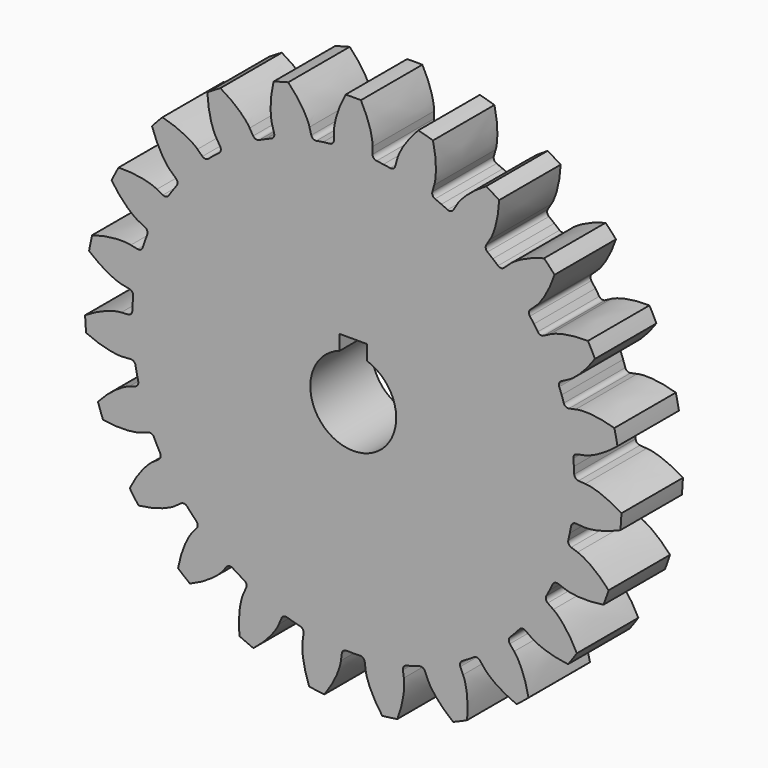
from build123d import *

# Parameters (mm, degrees)
F0_R     = 762
F1_DEPTH = 431.8


# Not quite as in the source:
# - ends of sketch curves that miss each other by under 0.0002 mm in the source are joined
# - the dataset's text gives a spline's control points without its knots; the knots are read off the source's solid


with BuildPart() as f1:
    # F0 (on Front) → F1 (new body)
    with BuildSketch(Plane.XZ):
        with BuildLine():
            ThreePointArc((207.1917137632, 1220.8943197928), (188.2251520352, 1223.9508569959), (169.2136060356, 1226.7138268041))
            ThreePointArc((169.2136060356, 1226.7138268041), (150.1616235918, 1229.1825683762), (131.0737537642, 1231.3564923478))
            ThreePointArc((131.0737537642, 1231.3564923478), (114.8688538687, 1239.6278770922), (108.3528186, 1256.6148096))
            Line((108.3528186, 1256.6148096), (108.3528186, 1294.8832116))
            add(Edge.make_bspline(
                [(42.8680118, 1503.1089826), (49.4976658, 1490.9197258), (64.0712968, 1462.3371058), (82.4042802, 1419.0365828), (96.2182734, 1376.5073308), (104.123363, 1342.6242388), (107.5962542, 1318.038004), (108.630847, 1303.1525118), (108.4084446, 1296.537158), (108.3528186, 1294.8832116)],
                knots=[7.154307, 7.154307, 7.154307, 7.154307, 8.792592, 10.941893, 12.700413, 14.068152, 15.04511, 15.631289, 15.826701, 15.826701, 15.826701, 15.826701], degree=3))
            ThreePointArc((42.8680118, 1503.1089826), (0, 1503.718354), (-42.8680115994, 1503.1089755464))
            add(Edge.make_bspline(
                [(-42.8680115994, 1503.1089755464), (-49.4976658, 1490.9197258), (-64.0712968, 1462.3371058), (-82.4042802, 1419.0365828), (-96.2182734, 1376.5073308), (-104.123363, 1342.6242388), (-107.5962542, 1318.038004), (-108.630847, 1303.1525118), (-108.4084446, 1296.537158), (-108.3528186, 1294.8832116)],
                knots=[7.154307, 7.154307, 7.154307, 7.154307, 8.792592, 10.941893, 12.700413, 14.068152, 15.04511, 15.631289, 15.826701, 15.826701, 15.826701, 15.826701], degree=3))
            Line((-108.3528186, 1294.8832116), (-108.3528186, 1256.6148096))
            ThreePointArc((-108.3528186, 1256.6148096), (-114.8688538687, 1239.6278770922), (-131.0737537202, 1231.3564919329))
            ThreePointArc((-131.0737537202, 1231.3564919329), (-150.1616235918, 1229.1825683762), (-169.2136060356, 1226.7138268041))
            ThreePointArc((-169.2136060356, 1226.7138268041), (-188.2251520352, 1223.9508569959), (-207.1917137632, 1220.8943197928))
            ThreePointArc((-207.1917137632, 1220.8943197928), (-225.0272880967, 1224.4869450629), (-235.884706456, 1239.0859614781))
            Line((-235.884706456, 1239.0859614781), (-246.2093882, 1275.9352688))
            add(Edge.make_bspline(
                [(-365.4445066, 1458.7718602), (-355.7720596, 1448.8232898), (-334.0273482, 1425.2325064), (-304.6918976, 1388.4838626), (-279.9158994, 1351.258664), (-263.1623896, 1320.764821), (-253.1850156, 1298.0272998), (-248.1727066, 1283.972921), (-246.6020722, 1277.5428856), (-246.2093882, 1275.9352688)],
                knots=[7.154307, 7.154307, 7.154307, 7.154307, 8.792592, 10.941893, 12.700413, 14.068152, 15.04511, 15.631289, 15.826701, 15.826701, 15.826701, 15.826701], degree=3))
            ThreePointArc((-365.4445066, 1458.7718602), (-406.8872538926, 1447.7929884321), (-448.001185685, 1435.6405592158))
            add(Edge.make_bspline(
                [(-448.001185685, 1435.6405592158), (-451.0964054, 1422.1146564), (-457.4181098, 1390.660033), (-463.3888878, 1344.019029), (-465.216367, 1299.339921), (-463.686779, 1264.580529), (-460.3975806, 1239.969072), (-457.3777746, 1225.3564266), (-455.3787946, 1219.0463808), (-454.8790242, 1217.4687614)],
                knots=[7.154307, 7.154307, 7.154307, 7.154307, 8.792592, 10.941893, 12.700413, 14.068152, 15.04511, 15.631289, 15.826701, 15.826701, 15.826701, 15.826701], degree=3))
            Line((-454.8790242, 1217.4687614), (-444.5543306, 1180.6194574))
            ThreePointArc((-444.5543306, 1180.6194574), (-446.2457074648, 1162.5044593237), (-459.6180792046, 1150.1677764018))
            ThreePointArc((-459.6180792046, 1150.1677764018), (-477.4116048133, 1142.924615064), (-495.0910348076, 1135.4072555989))
            ThreePointArc((-495.0910348076, 1135.4072555989), (-512.6521460867, 1127.6174880792), (-530.0907376222, 1119.5571758876))
            ThreePointArc((-530.0907376222, 1119.5571758876), (-548.2341895487, 1118.2046140224), (-562.6277429952, 1129.332952857))
            Line((-562.6277429952, 1129.332952857), (-582.5113826, 1162.0302134))
            add(Edge.make_bspline(
                [(-746.6536756, 1305.9174796), (-734.6558078, 1298.9474148), (-707.3527382, 1282.0980962), (-669.190432, 1254.6268024), (-635.2899918, 1225.4665102), (-610.9306044, 1200.6235068), (-595.1887004, 1181.4210306), (-586.570455, 1169.2401304), (-583.3232428, 1163.472273), (-582.5113826, 1162.0302134)],
                knots=[7.154307, 7.154307, 7.154307, 7.154307, 8.792592, 10.941893, 12.700413, 14.068152, 15.04511, 15.631289, 15.826701, 15.826701, 15.826701, 15.826701], degree=3))
            ThreePointArc((-746.6536756, 1305.9174796), (-783.5975441911, 1284.1646187591), (-819.9081683383, 1261.3704319712))
            add(Edge.make_bspline(
                [(-819.9081683383, 1261.3704319712), (-819.2393572, 1247.5110178), (-816.8402764, 1215.517254), (-810.0060762, 1168.9949442), (-799.7114816, 1125.479588), (-788.8606524, 1092.4218436), (-779.0533314, 1069.6104592), (-772.203053, 1056.3544278), (-768.575806, 1050.8177104), (-767.6689244, 1049.4334358)],
                knots=[7.154307, 7.154307, 7.154307, 7.154307, 8.792592, 10.941893, 12.700413, 14.068152, 15.04511, 15.631289, 15.826701, 15.826701, 15.826701, 15.826701], degree=3))
            Line((-767.6689244, 1049.4334358), (-747.785271, 1016.7361682))
            ThreePointArc((-747.785271, 1016.7361682), (-744.5265483812, 998.8365845229), (-754.0746415401, 983.3495450455))
            ThreePointArc((-754.0746415401, 983.3495450455), (-769.2541625123, 971.5743458654), (-784.2498366521, 959.5658934098))
            ThreePointArc((-784.2498366521, 959.5658934098), (-799.0580687681, 947.3270697848), (-813.6753327189, 934.8607897976))
            ThreePointArc((-813.6753327189, 934.8607897976), (-830.7810656895, 928.6633348644), (-847.6432640421, 935.49566387))
            Line((-847.6432640421, 935.49566387), (-875.6111774, 961.6158822))
            add(Edge.make_bspline(
                [(-1072.486933, 1055.8823688), (-1059.053508, 1052.4077504), (-1028.217019, 1043.5495258), (-984.0582046, 1027.3930176), (-943.547516, 1008.4602894), (-913.3888768, 991.1106162), (-893.0499538, 976.8673122), (-881.4649376, 967.4632924), (-876.7820158, 962.7854252), (-875.6111774, 961.6158822)],
                knots=[7.154307, 7.154307, 7.154307, 7.154307, 8.792592, 10.941893, 12.700413, 14.068152, 15.04511, 15.631289, 15.826701, 15.826701, 15.826701, 15.826701], degree=3))
            ThreePointArc((-1072.486933, 1055.8823688), (-1102.1919871804, 1024.9688146655), (-1131.0063300048, 993.2233942023))
            add(Edge.make_bspline(
                [(-1131.0063300048, 993.2233942023), (-1126.623096, 980.0583904), (-1115.681157, 949.8983034), (-1096.5488102, 906.9449984), (-1074.8956658, 867.8207688), (-1055.5283436, 838.916407), (-1039.9302798, 819.596913), (-1029.7575798, 808.680628), (-1024.7710518, 804.3278554), (-1023.5243182, 803.2395924)],
                knots=[7.154307, 7.154307, 7.154307, 7.154307, 8.792592, 10.941893, 12.700413, 14.068152, 15.04511, 15.631289, 15.826701, 15.826701, 15.826701, 15.826701], degree=3))
            Line((-1023.5243182, 803.2395924), (-995.5564036, 777.1193754))
            ThreePointArc((-995.5564036, 777.1193754), (-987.5892794345, 760.7627410412), (-992.6049562675, 743.2739570743))
            ThreePointArc((-992.6049562675, 743.2739570743), (-1004.0446531194, 727.8400320856), (-1015.244398185, 712.2311111541))
            ThreePointArc((-1015.244398185, 712.2311111541), (-1026.2015132755, 696.4509124069), (-1036.9133744925, 680.5032143638))
            ThreePointArc((-1036.9133744925, 680.5032143638), (-1051.7127205279, 669.9205067122), (-1069.7929606689, 671.9501118353))
            Line((-1069.7929606689, 671.9501118353), (-1103.7709192, 689.5560758))
            add(Edge.make_bspline(
                [(-1318.7787696, 727.2104582), (-1304.9060262, 727.4889946), (-1272.8231338, 727.278835), (-1225.9428872, 723.6353574), (-1181.82644, 716.334356), (-1148.1052984, 707.764777), (-1124.6777862, 699.5370312), (-1110.985205, 693.6073504), (-1105.2138424, 690.3663612), (-1103.7709192, 689.5560758)],
                knots=[7.154307, 7.154307, 7.154307, 7.154307, 8.792592, 10.941893, 12.700413, 14.068152, 15.04511, 15.631289, 15.826701, 15.826701, 15.826701, 15.826701], degree=3))
            ThreePointArc((-1318.7787696, 727.2104582), (-1339.0418965789, 689.4289359871), (-1358.2229115881, 651.0867087047))
            add(Edge.make_bspline(
                [(-1358.2229115881, 651.0867087047), (-1350.4503344, 639.5924724), (-1331.7770672, 613.5029132), (-1301.7655194, 577.304281), (-1270.3597656, 545.4728232), (-1243.9123204, 522.8655786), (-1223.6803314, 508.470789), (-1210.9397168, 500.7038754), (-1204.9637064, 497.8578562), (-1203.4696022, 497.146326)],
                knots=[7.154307, 7.154307, 7.154307, 7.154307, 8.792592, 10.941893, 12.700413, 14.068152, 15.04511, 15.631289, 15.826701, 15.826701, 15.826701, 15.826701], degree=3))
            Line((-1203.4696022, 497.146326), (-1169.4916666, 479.5403668))
            ThreePointArc((-1169.4916666, 479.5403668), (-1157.4070195713, 465.9397877294), (-1157.5182855896, 447.7463236647))
            ThreePointArc((-1157.5182855896, 447.7463236647), (-1164.3697442422, 429.7983306164), (-1170.9429379142, 411.7465699841))
            ThreePointArc((-1170.9429379142, 411.7465699841), (-1177.2362828369, 393.5953607754), (-1183.248278145, 375.3490324195))
            ThreePointArc((-1183.248278145, 375.3490324195), (-1194.6436427881, 361.1659361482), (-1212.6010042574, 358.242283599))
            Line((-1212.6010042574, 358.242283599), (-1250.0689756, 366.028224))
            add(Edge.make_bspline(
                [(-1467.2628008, 344.2778484), (-1453.9796676, 348.2888894), (-1423.0297676, 356.7423904), (-1376.9049678, 365.8821486), (-1332.4547138, 370.7543766), (-1297.6719792, 371.6004252), (-1272.8934156, 369.9984472), (-1258.1087614, 367.9828556), (-1251.6770242, 366.4191808), (-1250.0689756, 366.028224)],
                knots=[7.154307, 7.154307, 7.154307, 7.154307, 8.792592, 10.941893, 12.700413, 14.068152, 15.04511, 15.631289, 15.826701, 15.826701, 15.826701, 15.826701], degree=3))
            ThreePointArc((-1467.2628008, 344.2778484), (-1476.5811900429, 302.4304522076), (-1484.7063103238, 260.3350917556))
            add(Edge.make_bspline(
                [(-1484.7063103238, 260.3350917556), (-1474.1208516, 251.364115), (-1449.1011658, 231.2800048), (-1410.4362698, 204.5207238), (-1371.6070866, 182.3428408), (-1340.0410334, 167.709342), (-1316.6756242, 159.306895), (-1302.311975, 155.2653994), (-1295.7897376, 154.1372076), (-1294.1590576, 153.855166)],
                knots=[7.154307, 7.154307, 7.154307, 7.154307, 8.792592, 10.941893, 12.700413, 14.068152, 15.04511, 15.631289, 15.826701, 15.826701, 15.826701, 15.826701], degree=3))
            Line((-1294.1590576, 153.855166), (-1256.6910858, 146.0692278))
            ThreePointArc((-1256.6910858, 146.0692278), (-1241.385179011, 136.233393155), (-1236.5837786479, 118.6845752562))
            ThreePointArc((-1236.5837786479, 118.6845752562), (-1238.3388559954, 99.5536385174), (-1239.7979913123, 80.3978572005))
            ThreePointArc((-1239.7979913123, 80.3978572005), (-1240.9608244985, 61.221816461), (-1241.8270783309, 42.0300910628))
            ThreePointArc((-1241.8270783309, 42.0300910628), (-1248.9733177093, 25.298515831), (-1265.4759809502, 17.6384509204))
            Line((-1265.4759809502, 17.6384509204), (-1303.6551778, 15.0269194))
            add(Edge.make_bspline(
                [(-1506.9266788, -64.5150856), (-1495.2182694, -57.0690502), (-1467.6968106, -40.5788368), (-1425.7483296, -19.3336672), (-1384.2609094, -2.649601), (-1350.996282, 7.5493626), (-1326.704357, 12.6919482), (-1311.9241732, 14.7399756), (-1305.3090734, 14.9695154), (-1303.6551778, 15.0269194)],
                knots=[7.154307, 7.154307, 7.154307, 7.154307, 8.792592, 10.941893, 12.700413, 14.068152, 15.04511, 15.631289, 15.826701, 15.826701, 15.826701, 15.826701], degree=3))
            ThreePointArc((-1506.9266788, -64.5150856), (-1504.6092126713, -107.3247336701), (-1501.0758396072, -150.0512112007))
            add(Edge.make_bspline(
                [(-1501.0758396072, -150.0512112007), (-1488.4625806, -155.8336228), (-1458.9520478, -168.4227264), (-1414.5013874, -183.7580272), (-1371.128576, -194.6375076), (-1336.7850074, -200.2119186), (-1312.0191184, -201.9988848), (-1297.0977106, -202.0152424), (-1290.5129638, -201.3419138), (-1288.8666628, -201.1735626)],
                knots=[7.154307, 7.154307, 7.154307, 7.154307, 8.792592, 10.941893, 12.700413, 14.068152, 15.04511, 15.631289, 15.826701, 15.826701, 15.826701, 15.826701], degree=3))
            Line((-1288.8666628, -201.1735626), (-1250.6874656, -198.5620362))
            ThreePointArc((-1250.6874656, -198.5620362), (-1233.2954715893, -203.903634229), (-1223.9375104416, -219.5062927103))
            ThreePointArc((-1223.9375104416, -219.5062927103), (-1220.4660423092, -238.4013096037), (-1216.7029025722, -257.2404054098))
            ThreePointArc((-1216.7029025722, -257.2404054098), (-1212.6489780375, -276.0190888106), (-1208.3052400256, -294.7328589942))
            ThreePointArc((-1208.3052400256, -294.7328589942), (-1210.6723585001, -312.7720099861), (-1224.4963843289, -324.6003873353))
            Line((-1224.4963843289, -324.6003873353), (-1260.5552132, -337.4156828))
            add(Edge.make_bspline(
                [(-1434.8286772, -468.8500402), (-1425.5633668, -458.5212318), (-1403.5114932, -435.2173414), (-1368.85045, -403.442424), (-1333.4028196, -376.1838806), (-1304.1233506, -357.3884394), (-1282.1197116, -345.8826712), (-1268.4401606, -339.9229422), (-1262.1322992, -337.9171804), (-1260.5552132, -337.4156828)],
                knots=[7.154307, 7.154307, 7.154307, 7.154307, 8.792592, 10.941893, 12.700413, 14.068152, 15.04511, 15.631289, 15.826701, 15.826701, 15.826701, 15.826701], degree=3))
            ThreePointArc((-1434.8286772, -468.8500402), (-1421.0472548272, -509.4469564436), (-1406.1174406458, -549.6357343076))
            add(Edge.make_bspline(
                [(-1406.1174406458, -549.6357343076), (-1392.4118456, -551.8006744), (-1360.5991584, -555.9611182), (-1313.659425, -558.735103), (-1268.959743, -557.509299), (-1234.385771, -553.6112118), (-1210.056127, -548.6501346), (-1195.6836386, -544.6401604), (-1189.5247482, -542.2152478), (-1187.9848986, -541.6089752)],
                knots=[7.154307, 7.154307, 7.154307, 7.154307, 8.792592, 10.941893, 12.700413, 14.068152, 15.04511, 15.631289, 15.826701, 15.826701, 15.826701, 15.826701], degree=3))
            Line((-1187.9848986, -541.6089752), (-1151.9260934, -528.7936592))
            ThreePointArc((-1151.9260934, -528.7936592), (-1133.7378843182, -529.2448847468), (-1120.5173863074, -541.7442014947))
            ThreePointArc((-1120.5173863074, -541.7442014947), (-1112.0768418425, -559.0019586944), (-1103.3705195132, -576.127171864))
            ThreePointArc((-1103.3705195132, -576.127171864), (-1094.4005004888, -593.1157486601), (-1085.1689286269, -609.9636287587))
            ThreePointArc((-1085.1689286269, -609.9636287587), (-1082.5813731463, -627.9724758858), (-1092.7015046064, -643.0918966742))
            Line((-1092.7015046064, -643.0918966742), (-1123.9656464, -665.1605442))
            add(Edge.make_bspline(
                [(-1256.316004, -838.739369), (-1250.1809642, -826.2938262), (-1235.2341564, -797.9045764), (-1210.4311834, -757.9565232), (-1183.652319, -722.1451394), (-1160.5295814, -696.147198), (-1142.4461022, -679.1315602), (-1130.8817362, -669.7021404), (-1125.3489304, -666.068899), (-1123.9656464, -665.1605442)],
                knots=[7.154307, 7.154307, 7.154307, 7.154307, 8.792592, 10.941893, 12.700413, 14.068152, 15.04511, 15.631289, 15.826701, 15.826701, 15.826701, 15.826701], degree=3))
            ThreePointArc((-1256.316004, -838.739369), (-1232.0927158282, -874.1126625528), (-1206.8737342356, -908.7831191776))
            add(Edge.make_bspline(
                [(-1206.8737342356, -908.7831191776), (-1193.0922798, -907.1700424), (-1161.3368188, -902.5932418), (-1115.3893364, -892.6001706), (-1072.6779664, -879.3599888), (-1040.4377718, -866.2785062), (-1018.3488396, -854.9373554), (-1005.5911816, -847.1984326), (-1000.3149158, -843.201768), (-998.9957414, -842.202532)],
                knots=[7.154307, 7.154307, 7.154307, 7.154307, 8.792592, 10.941893, 12.700413, 14.068152, 15.04511, 15.631289, 15.826701, 15.826701, 15.826701, 15.826701], degree=3))
            Line((-998.9957414, -842.202532), (-967.731618, -820.1338944))
            ThreePointArc((-967.731618, -820.1338944), (-950.0961395823, -815.6612726178), (-933.9936239178, -824.1302434205))
            ThreePointArc((-933.9936239178, -824.1302434205), (-921.2099913722, -838.4708010991), (-908.2061979962, -852.6120249892))
            ThreePointArc((-908.2061979962, -852.6120249892), (-894.9853513159, -866.5505341967), (-881.5506104913, -880.2829980997))
            ThreePointArc((-881.5506104913, -880.2829980997), (-874.2002628674, -896.9259218018), (-879.8659530492, -914.2150656515))
            Line((-879.8659530492, -914.2150656515), (-904.0166832, -943.9002966))
            add(Edge.make_bspline(
                [(-984.6281298, -1146.750056), (-982.0783508, -1133.1108148), (-975.345141, -1101.7417132), (-962.2397824, -1056.5832818), (-946.1157608, -1014.875034), (-930.8646356, -983.6027064), (-918.0425124, -962.339198), (-909.4510132, -950.1394256), (-905.1036, -945.1481986), (-904.0166832, -943.9002966)],
                knots=[7.154307, 7.154307, 7.154307, 7.154307, 8.792592, 10.941893, 12.700413, 14.068152, 15.04511, 15.631289, 15.826701, 15.826701, 15.826701, 15.826701], degree=3))
            ThreePointArc((-984.6281298, -1146.750056), (-951.7595055841, -1174.2762366618), (-918.121739889, -1200.8570153711))
            add(Edge.make_bspline(
                [(-918.121739889, -1200.8570153711), (-905.2865308, -1195.5855692), (-875.9434602, -1182.6109698), (-834.3959436, -1160.5919892), (-796.8405704, -1136.3193936), (-769.3252838, -1115.0247194), (-751.1152618, -1098.1445906), (-740.918635, -1087.250683), (-736.9163062, -1081.9787098), (-735.9156478, -1080.6606276)],
                knots=[7.154307, 7.154307, 7.154307, 7.154307, 8.792592, 10.941893, 12.700413, 14.068152, 15.04511, 15.631289, 15.826701, 15.826701, 15.826701, 15.826701], degree=3))
            Line((-735.9156478, -1080.6606276), (-711.7649214, -1050.9753936))
            ThreePointArc((-711.7649214, -1050.9753936), (-695.9901259568, -1041.9106321688), (-678.1998408489, -1045.7211294955))
            ThreePointArc((-678.1998408489, -1045.7211294955), (-662.0212203823, -1056.0809143876), (-645.6843854666, -1066.1893626561))
            ThreePointArc((-645.6843854666, -1066.1893626561), (-629.193233555, -1076.0440557024), (-612.5517095331, -1085.6426360471))
            ThreePointArc((-612.5517095331, -1085.6426360471), (-600.9837283129, -1099.6853020294), (-601.7747607234, -1117.8619025607))
            Line((-601.7747607234, -1117.8619025607), (-617.0209402, -1152.9621086))
            add(Edge.make_bspline(
                [(-639.9148746, -1370.0383572), (-641.1394848, -1356.2169726), (-643.119237, -1324.1945068), (-642.6834746, -1277.1749158), (-638.4101024, -1232.6630922), (-632.1617024, -1198.4357286), (-625.5518858, -1174.5013848), (-620.5704378, -1160.4360332), (-617.7308702, -1154.4569748), (-617.0209402, -1152.9621086)],
                knots=[7.154307, 7.154307, 7.154307, 7.154307, 8.792592, 10.941893, 12.700413, 14.068152, 15.04511, 15.631289, 15.826701, 15.826701, 15.826701, 15.826701], degree=3))
            ThreePointArc((-639.9148746, -1370.0383572), (-600.8386419489, -1387.6759408107), (-561.2768558469, -1404.1956682157))
            add(Edge.make_bspline(
                [(-561.2768558469, -1404.1956682157), (-550.3398188, -1395.6568226), (-525.5853852, -1375.246678), (-491.51921, -1342.8348048), (-461.9051468, -1309.3300204), (-441.1554296, -1281.4014504), (-428.174912, -1260.2343096), (-421.2955506, -1246.9933404), (-418.8639832, -1240.8370408), (-418.2560596, -1239.297877)],
                knots=[7.154307, 7.154307, 7.154307, 7.154307, 8.792592, 10.941893, 12.700413, 14.068152, 15.04511, 15.631289, 15.826701, 15.826701, 15.826701, 15.826701], degree=3))
            Line((-418.2560596, -1239.297877), (-403.0098874, -1204.1976678))
            ThreePointArc((-403.0098874, -1204.1976678), (-390.2656925401, -1191.2130621309), (-372.1070557635, -1190.0824882937))
            ThreePointArc((-372.1070557635, -1190.0824882937), (-353.7333473791, -1195.6931698795), (-335.275099724, -1201.019144067))
            ThreePointArc((-335.275099724, -1201.019144067), (-316.7367201822, -1206.0591386589), (-298.1226431187, -1210.8119479964))
            ThreePointArc((-298.1226431187, -1210.8119479964), (-283.1949670005, -1221.2128578376), (-279.0526829476, -1238.9288400498))
            Line((-279.0526829476, -1238.9288400498), (-284.2635666, -1276.8408042))
            add(Edge.make_bspline(
                [(-247.742075, -1492.0439806), (-252.650244, -1479.0655458), (-263.1961208, -1448.764692), (-275.4622634, -1403.3711328), (-283.3565072, -1359.3569968), (-286.57423, -1324.7130732), (-286.66694, -1299.882973), (-285.6650116, -1284.9952456), (-284.543881, -1278.471789), (-284.2635666, -1276.8408042)],
                knots=[7.154307, 7.154307, 7.154307, 7.154307, 8.792592, 10.941893, 12.700413, 14.068152, 15.04511, 15.631289, 15.826701, 15.826701, 15.826701, 15.826701], degree=3))
            ThreePointArc((-247.742075, -1492.0439806), (-205.3563291936, -1498.4848881564), (-162.8046272215, -1503.7183777557))
            add(Edge.make_bspline(
                [(-162.8046272215, -1503.7183777557), (-154.5769324, -1492.545402), (-136.2470478, -1466.2134506), (-112.1887266, -1425.8125662), (-92.7123622, -1385.5604242), (-80.2671242, -1353.0693284), (-73.478771, -1329.1849972), (-70.4268848, -1314.579032), (-69.7464442, -1307.9949964), (-69.576315, -1306.3488986)],
                knots=[7.154307, 7.154307, 7.154307, 7.154307, 8.792592, 10.941893, 12.700413, 14.068152, 15.04511, 15.631289, 15.826701, 15.826701, 15.826701, 15.826701], degree=3))
            Line((-69.576315, -1306.3488986), (-64.3654288, -1268.4369094))
            ThreePointArc((-64.3654288, -1268.4369094), (-55.5970452045, -1252.4954617702), (-38.4167887865, -1246.5076919647))
            ThreePointArc((-38.4167887865, -1246.5076919647), (-19.2106900217, -1246.9531491193), (0, -1247.101646))
            ThreePointArc((0, -1247.101646), (19.2106900217, -1246.9531491193), (38.4167888485, -1246.5076939665))
            ThreePointArc((38.4167888485, -1246.5076939665), (55.5970452045, -1252.4954617702), (64.3654511814, -1268.4369063237))
            Line((64.3654511814, -1268.4369063237), (69.576315, -1306.3488986))
            add(Edge.make_bspline(
                [(162.8046274, -1503.7183794), (154.5769324, -1492.545402), (136.2470478, -1466.2134506), (112.1887266, -1425.8125662), (92.7123622, -1385.5604242), (80.2671242, -1353.0693284), (73.478771, -1329.1849972), (70.4268848, -1314.579032), (69.7464442, -1307.9949964), (69.576315, -1306.3488986)],
                knots=[7.154307, 7.154307, 7.154307, 7.154307, 8.792592, 10.941893, 12.700413, 14.068152, 15.04511, 15.631289, 15.826701, 15.826701, 15.826701, 15.826701], degree=3))
            ThreePointArc((162.8046274, -1503.7183794), (205.3563291936, -1498.4848881564), (247.7420772114, -1492.0439938788))
            add(Edge.make_bspline(
                [(247.7420772114, -1492.0439938788), (252.650244, -1479.0655458), (263.1961208, -1448.764692), (275.4622634, -1403.3711328), (283.3565072, -1359.3569968), (286.57423, -1324.7130732), (286.66694, -1299.882973), (285.6650116, -1284.9952456), (284.543881, -1278.471789), (284.2635666, -1276.8408042)],
                knots=[7.154307, 7.154307, 7.154307, 7.154307, 8.792592, 10.941893, 12.700413, 14.068152, 15.04511, 15.631289, 15.826701, 15.826701, 15.826701, 15.826701], degree=3))
            Line((284.2635666, -1276.8408042), (279.0526804, -1238.9288404))
            ThreePointArc((279.0526804, -1238.9288404), (283.1949670005, -1221.2128578376), (298.1226412207, -1210.8119403158))
            ThreePointArc((298.1226412207, -1210.8119403158), (316.7367201822, -1206.0591386589), (335.275099724, -1201.019144067))
            ThreePointArc((335.275099724, -1201.019144067), (353.7333473791, -1195.6931698795), (372.1070556523, -1190.0824879394))
            ThreePointArc((372.1070556523, -1190.0824879394), (390.2656925401, -1191.2130621309), (403.0098733082, -1204.1976739209))
            Line((403.0098733082, -1204.1976739209), (418.2560596, -1239.297877))
            add(Edge.make_bspline(
                [(561.2768556, -1404.1956676), (550.3398188, -1395.6568226), (525.5853852, -1375.246678), (491.51921, -1342.8348048), (461.9051468, -1309.3300204), (441.1554296, -1281.4014504), (428.174912, -1260.2343096), (421.2955506, -1246.9933404), (418.8639832, -1240.8370408), (418.2560596, -1239.297877)],
                knots=[7.154307, 7.154307, 7.154307, 7.154307, 8.792592, 10.941893, 12.700413, 14.068152, 15.04511, 15.631289, 15.826701, 15.826701, 15.826701, 15.826701], degree=3))
            ThreePointArc((561.2768556, -1404.1956676), (600.8386419489, -1387.6759408107), (639.9148743546, -1370.0383566763))
            add(Edge.make_bspline(
                [(639.9148743546, -1370.0383566763), (641.1394848, -1356.2169726), (643.119237, -1324.1945068), (642.6834746, -1277.1749158), (638.4101024, -1232.6630922), (632.1617024, -1198.4357286), (625.5518858, -1174.5013848), (620.5704378, -1160.4360332), (617.7308702, -1154.4569748), (617.0209402, -1152.9621086)],
                knots=[7.154307, 7.154307, 7.154307, 7.154307, 8.792592, 10.941893, 12.700413, 14.068152, 15.04511, 15.631289, 15.826701, 15.826701, 15.826701, 15.826701], degree=3))
            Line((617.0209402, -1152.9621086), (601.774768, -1117.8618994))
            ThreePointArc((601.774768, -1117.8618994), (600.9837283129, -1099.6853020294), (612.551714006, -1085.6426439423))
            ThreePointArc((612.551714006, -1085.6426439423), (629.193233555, -1076.0440557024), (645.6843854666, -1066.1893626561))
            ThreePointArc((645.6843854666, -1066.1893626561), (662.0212203823, -1056.0809143876), (678.1998376342, -1045.7211245596))
            ThreePointArc((678.1998376342, -1045.7211245596), (695.9901259568, -1041.9106321688), (711.7649251508, -1050.9753905485))
            Line((711.7649251508, -1050.9753905485), (735.9156478, -1080.6606276))
            add(Edge.make_bspline(
                [(918.121735, -1200.857009), (905.2865308, -1195.5855692), (875.9434602, -1182.6109698), (834.3959436, -1160.5919892), (796.8405704, -1136.3193936), (769.3252838, -1115.0247194), (751.1152618, -1098.1445906), (740.918635, -1087.250683), (736.9163062, -1081.9787098), (735.9156478, -1080.6606276)],
                knots=[7.154307, 7.154307, 7.154307, 7.154307, 8.792592, 10.941893, 12.700413, 14.068152, 15.04511, 15.631289, 15.826701, 15.826701, 15.826701, 15.826701], degree=3))
            ThreePointArc((918.121735, -1200.857009), (951.7595055841, -1174.2762366618), (984.6281287742, -1146.7500548099))
            add(Edge.make_bspline(
                [(984.6281287742, -1146.7500548099), (982.0783508, -1133.1108148), (975.345141, -1101.7417132), (962.2397824, -1056.5832818), (946.1157608, -1014.875034), (930.8646356, -983.6027064), (918.0425124, -962.339198), (909.4510132, -950.1394256), (905.1036, -945.1481986), (904.0166832, -943.9002966)],
                knots=[7.154307, 7.154307, 7.154307, 7.154307, 8.792592, 10.941893, 12.700413, 14.068152, 15.04511, 15.631289, 15.826701, 15.826701, 15.826701, 15.826701], degree=3))
            Line((904.0166832, -943.9002966), (879.8659568, -914.2150626))
            ThreePointArc((879.8659568, -914.2150626), (874.2002628674, -896.9259218018), (881.5506093621, -880.2829969778))
            ThreePointArc((881.5506093621, -880.2829969778), (894.9853513159, -866.5505341967), (908.2061979962, -852.6120249892))
            ThreePointArc((908.2061979962, -852.6120249892), (921.2099913722, -838.4708010991), (933.9936231128, -824.1302427139))
            ThreePointArc((933.9936231128, -824.1302427139), (950.0961395823, -815.6612726178), (967.7316194406, -820.1338923591))
            Line((967.7316194406, -820.1338923591), (998.9957414, -842.202532))
            add(Edge.make_bspline(
                [(1206.8737356, -908.7831202), (1193.0922798, -907.1700424), (1161.3368188, -902.5932418), (1115.3893364, -892.6001706), (1072.6779664, -879.3599888), (1040.4377718, -866.2785062), (1018.3488396, -854.9373554), (1005.5911816, -847.1984326), (1000.3149158, -843.201768), (998.9957414, -842.202532)],
                knots=[7.154307, 7.154307, 7.154307, 7.154307, 8.792592, 10.941893, 12.700413, 14.068152, 15.04511, 15.631289, 15.826701, 15.826701, 15.826701, 15.826701], degree=3))
            ThreePointArc((1206.8737356, -908.7831202), (1232.0927158282, -874.1126625528), (1256.3160098136, -838.7393728609))
            add(Edge.make_bspline(
                [(1256.3160098136, -838.7393728609), (1250.1809642, -826.2938262), (1235.2341564, -797.9045764), (1210.4311834, -757.9565232), (1183.652319, -722.1451394), (1160.5295814, -696.147198), (1142.4461022, -679.1315602), (1130.8817362, -669.7021404), (1125.3489304, -666.068899), (1123.9656464, -665.1605442)],
                knots=[7.154307, 7.154307, 7.154307, 7.154307, 8.792592, 10.941893, 12.700413, 14.068152, 15.04511, 15.631289, 15.826701, 15.826701, 15.826701, 15.826701], degree=3))
            Line((1123.9656464, -665.1605442), (1092.7014976, -643.0919066))
            ThreePointArc((1092.7014976, -643.0919066), (1082.5813731463, -627.9724758858), (1085.1689334825, -609.9636314683))
            ThreePointArc((1085.1689334825, -609.9636314683), (1094.4005004888, -593.1157486601), (1103.3705195132, -576.127171864))
            ThreePointArc((1103.3705195132, -576.127171864), (1112.0768418425, -559.0019586944), (1120.5173868381, -541.7442017492))
            ThreePointArc((1120.5173868381, -541.7442017492), (1133.7378843182, -529.2448847468), (1151.9260916711, -528.7936640647))
            Line((1151.9260916711, -528.7936640647), (1187.9848986, -541.6089752))
            add(Edge.make_bspline(
                [(1406.1174316, -549.6357308), (1392.4118456, -551.8006744), (1360.5991584, -555.9611182), (1313.659425, -558.735103), (1268.959743, -557.509299), (1234.385771, -553.6112118), (1210.056127, -548.6501346), (1195.6836386, -544.6401604), (1189.5247482, -542.2152478), (1187.9848986, -541.6089752)],
                knots=[7.154307, 7.154307, 7.154307, 7.154307, 8.792592, 10.941893, 12.700413, 14.068152, 15.04511, 15.631289, 15.826701, 15.826701, 15.826701, 15.826701], degree=3))
            ThreePointArc((1406.1174316, -549.6357308), (1421.0472548272, -509.4469564436), (1434.8286823394, -468.8500418636))
            add(Edge.make_bspline(
                [(1434.8286823394, -468.8500418636), (1425.5633668, -458.5212318), (1403.5114932, -435.2173414), (1368.85045, -403.442424), (1333.4028196, -376.1838806), (1304.1233506, -357.3884394), (1282.1197116, -345.8826712), (1268.4401606, -339.9229422), (1262.1322992, -337.9171804), (1260.5552132, -337.4156828)],
                knots=[7.154307, 7.154307, 7.154307, 7.154307, 8.792592, 10.941893, 12.700413, 14.068152, 15.04511, 15.631289, 15.826701, 15.826701, 15.826701, 15.826701], degree=3))
            Line((1260.5552132, -337.4156828), (1224.4963826, -324.6003922))
            ThreePointArc((1224.4963826, -324.6003922), (1210.6723585001, -312.7720099861), (1208.3052413347, -294.7328593088))
            ThreePointArc((1208.3052413347, -294.7328593088), (1212.6489780375, -276.0190888106), (1216.7029025722, -257.2404054098))
            ThreePointArc((1216.7029025722, -257.2404054098), (1220.4660423092, -238.4013096037), (1223.9375007503, -219.5062910071))
            ThreePointArc((1223.9375007503, -219.5062910071), (1233.2954715893, -203.903634229), (1250.6874669791, -198.5620160387))
            Line((1250.6874669791, -198.5620160387), (1288.8666628, -201.1735626))
            add(Edge.make_bspline(
                [(1501.0758396, -150.0512112), (1488.4625806, -155.8336228), (1458.9520478, -168.4227264), (1414.5013874, -183.7580272), (1371.128576, -194.6375076), (1336.7850074, -200.2119186), (1312.0191184, -201.9988848), (1297.0977106, -202.0152424), (1290.5129638, -201.3419138), (1288.8666628, -201.1735626)],
                knots=[7.154307, 7.154307, 7.154307, 7.154307, 8.792592, 10.941893, 12.700413, 14.068152, 15.04511, 15.631289, 15.826701, 15.826701, 15.826701, 15.826701], degree=3))
            ThreePointArc((1501.0758396, -150.0512112), (1504.6092126713, -107.3247336701), (1506.9266707946, -64.5150852807))
            add(Edge.make_bspline(
                [(1506.9266707946, -64.5150852807), (1495.2182694, -57.0690502), (1467.6968106, -40.5788368), (1425.7483296, -19.3336672), (1384.2609094, -2.649601), (1350.996282, 7.5493626), (1326.704357, 12.6919482), (1311.9241732, 14.7399756), (1305.3090734, 14.9695154), (1303.6551778, 15.0269194)],
                knots=[7.154307, 7.154307, 7.154307, 7.154307, 8.792592, 10.941893, 12.700413, 14.068152, 15.04511, 15.631289, 15.826701, 15.826701, 15.826701, 15.826701], degree=3))
            Line((1303.6551778, 15.0269194), (1265.4759806, 17.6384458))
            ThreePointArc((1265.4759806, 17.6384458), (1248.9733177093, 25.298515831), (1241.8270674817, 42.0300906571))
            ThreePointArc((1241.8270674817, 42.0300906571), (1240.9608244985, 61.221816461), (1239.7979913123, 80.3978572005))
            ThreePointArc((1239.7979913123, 80.3978572005), (1238.3388559954, 99.5536385174), (1236.5837677015, 118.6845741666))
            ThreePointArc((1236.5837677015, 118.6845741666), (1241.385179011, 136.233393155), (1256.6910853426, 146.069230001))
            Line((1256.6910853426, 146.069230001), (1294.1590576, 153.855166))
            add(Edge.make_bspline(
                [(1484.7063016, 260.3350902), (1474.1208516, 251.364115), (1449.1011658, 231.2800048), (1410.4362698, 204.5207238), (1371.6070866, 182.3428408), (1340.0410334, 167.709342), (1316.6756242, 159.306895), (1302.311975, 155.2653994), (1295.7897376, 154.1372076), (1294.1590576, 153.855166)],
                knots=[7.154307, 7.154307, 7.154307, 7.154307, 8.792592, 10.941893, 12.700413, 14.068152, 15.04511, 15.631289, 15.826701, 15.826701, 15.826701, 15.826701], degree=3))
            ThreePointArc((1484.7063016, 260.3350902), (1476.5811900429, 302.4304522076), (1467.2628047928, 344.2778493489))
            add(Edge.make_bspline(
                [(1467.2628047928, 344.2778493489), (1453.9796676, 348.2888894), (1423.0297676, 356.7423904), (1376.9049678, 365.8821486), (1332.4547138, 370.7543766), (1297.6719792, 371.6004252), (1272.8934156, 369.9984472), (1258.1087614, 367.9828556), (1251.6770242, 366.4191808), (1250.0689756, 366.028224)],
                knots=[7.154307, 7.154307, 7.154307, 7.154307, 8.792592, 10.941893, 12.700413, 14.068152, 15.04511, 15.631289, 15.826701, 15.826701, 15.826701, 15.826701], degree=3))
            Line((1250.0689756, 366.028224), (1212.6010038, 358.2422858))
            ThreePointArc((1212.6010038, 358.2422858), (1194.6436427881, 361.1659361482), (1183.2482766855, 375.3490319511))
            ThreePointArc((1183.2482766855, 375.3490319511), (1177.2362828369, 393.5953607754), (1170.9429379142, 411.7465699841))
            ThreePointArc((1170.9429379142, 411.7465699841), (1164.3697442422, 429.7983306164), (1157.5182756859, 447.7463197961))
            ThreePointArc((1157.5182756859, 447.7463197961), (1157.4070195713, 465.9397877294), (1169.4916641311, 479.5403715647))
            Line((1169.4916641311, 479.5403715647), (1203.4696022, 497.146326))
            add(Edge.make_bspline(
                [(1358.2229122, 651.086709), (1350.4503344, 639.5924724), (1331.7770672, 613.5029132), (1301.7655194, 577.304281), (1270.3597656, 545.4728232), (1243.9123204, 522.8655786), (1223.6803314, 508.470789), (1210.9397168, 500.7038754), (1204.9637064, 497.8578562), (1203.4696022, 497.146326)],
                knots=[7.154307, 7.154307, 7.154307, 7.154307, 8.792592, 10.941893, 12.700413, 14.068152, 15.04511, 15.631289, 15.826701, 15.826701, 15.826701, 15.826701], degree=3))
            ThreePointArc((1358.2229122, 651.086709), (1339.0418965789, 689.4289359871), (1318.7787653439, 727.2104558388))
            add(Edge.make_bspline(
                [(1318.7787653439, 727.2104558388), (1304.9060262, 727.4889946), (1272.8231338, 727.278835), (1225.9428872, 723.6353574), (1181.82644, 716.334356), (1148.1052984, 707.764777), (1124.6777862, 699.5370312), (1110.985205, 693.6073504), (1105.2138424, 690.3663612), (1103.7709192, 689.5560758)],
                knots=[7.154307, 7.154307, 7.154307, 7.154307, 8.792592, 10.941893, 12.700413, 14.068152, 15.04511, 15.631289, 15.826701, 15.826701, 15.826701, 15.826701], degree=3))
            Line((1103.7709192, 689.5560758), (1069.7929582, 671.9501166))
            ThreePointArc((1069.7929582, 671.9501166), (1051.7127205279, 669.9205067122), (1036.9133721748, 680.5032128328))
            ThreePointArc((1036.9133721748, 680.5032128328), (1026.2015132755, 696.4509124069), (1015.244398185, 712.2311111541))
            ThreePointArc((1015.244398185, 712.2311111541), (1004.0446531194, 727.8400320856), (992.6049497129, 743.273952137))
            ThreePointArc((992.6049497129, 743.273952137), (987.5892794345, 760.7627410412), (995.5564023579, 777.11937673))
            Line((995.5564023579, 777.11937673), (1023.5243182, 803.2395924))
            add(Edge.make_bspline(
                [(1131.0063232, 993.2233882), (1126.623096, 980.0583904), (1115.681157, 949.8983034), (1096.5488102, 906.9449984), (1074.8956658, 867.8207688), (1055.5283436, 838.916407), (1039.9302798, 819.596913), (1029.7575798, 808.680628), (1024.7710518, 804.3278554), (1023.5243182, 803.2395924)],
                knots=[7.154307, 7.154307, 7.154307, 7.154307, 8.792592, 10.941893, 12.700413, 14.068152, 15.04511, 15.631289, 15.826701, 15.826701, 15.826701, 15.826701], degree=3))
            ThreePointArc((1131.0063232, 993.2233882), (1102.1919871804, 1024.9688146655), (1072.4869328264, 1055.8823686284))
            add(Edge.make_bspline(
                [(1072.4869328264, 1055.8823686284), (1059.053508, 1052.4077504), (1028.217019, 1043.5495258), (984.0582046, 1027.3930176), (943.547516, 1008.4602894), (913.3888768, 991.1106162), (893.0499538, 976.8673122), (881.4649376, 967.4632924), (876.7820158, 962.7854252), (875.6111774, 961.6158822)],
                knots=[7.154307, 7.154307, 7.154307, 7.154307, 8.792592, 10.941893, 12.700413, 14.068152, 15.04511, 15.631289, 15.826701, 15.826701, 15.826701, 15.826701], degree=3))
            Line((875.6111774, 961.6158822), (847.6432628, 935.4956652))
            ThreePointArc((847.6432628, 935.4956652), (830.7810656895, 928.6633348644), (813.6753375013, 934.8607953183))
            ThreePointArc((813.6753375013, 934.8607953183), (799.0580687681, 947.3270697848), (784.2498366521, 959.5658934098))
            ThreePointArc((784.2498366521, 959.5658934098), (769.2541625123, 971.5743458654), (754.0746427761, 983.3495466645))
            ThreePointArc((754.0746427761, 983.3495466645), (744.5265483812, 998.8365845229), (747.785264062, 1016.7361724191))
            Line((747.785264062, 1016.7361724191), (767.6689244, 1049.4334358))
            add(Edge.make_bspline(
                [(819.9081646, 1261.3704262), (819.2393572, 1247.5110178), (816.8402764, 1215.517254), (810.0060762, 1168.9949442), (799.7114816, 1125.479588), (788.8606524, 1092.4218436), (779.0533314, 1069.6104592), (772.203053, 1056.3544278), (768.575806, 1050.8177104), (767.6689244, 1049.4334358)],
                knots=[7.154307, 7.154307, 7.154307, 7.154307, 8.792592, 10.941893, 12.700413, 14.068152, 15.04511, 15.631289, 15.826701, 15.826701, 15.826701, 15.826701], degree=3))
            ThreePointArc((819.9081646, 1261.3704262), (783.5975441911, 1284.1646187591), (746.6536739928, 1305.9174767795))
            add(Edge.make_bspline(
                [(746.6536739928, 1305.9174767795), (734.6558078, 1298.9474148), (707.3527382, 1282.0980962), (669.190432, 1254.6268024), (635.2899918, 1225.4665102), (610.9306044, 1200.6235068), (595.1887004, 1181.4210306), (586.570455, 1169.2401304), (583.3232428, 1163.472273), (582.5113826, 1162.0302134)],
                knots=[7.154307, 7.154307, 7.154307, 7.154307, 8.792592, 10.941893, 12.700413, 14.068152, 15.04511, 15.631289, 15.826701, 15.826701, 15.826701, 15.826701], degree=3))
            Line((582.5113826, 1162.0302134), (562.6277546, 1129.3329458))
            ThreePointArc((562.6277546, 1129.3329458), (548.2341895487, 1118.2046140224), (530.0907364889, 1119.5571734847))
            ThreePointArc((530.0907364889, 1119.5571734847), (512.6521460867, 1127.6174880792), (495.0910348076, 1135.4072555989))
            ThreePointArc((495.0910348076, 1135.4072555989), (477.4116048133, 1142.924615064), (459.6180773338, 1150.1677717025))
            ThreePointArc((459.6180773338, 1150.1677717025), (446.2457074648, 1162.5044593237), (444.554318744, 1180.6194607219))
            Line((444.554318744, 1180.6194607219), (454.8790242, 1217.4687614))
            add(Edge.make_bspline(
                [(448.0011868, 1435.6405628), (451.0964054, 1422.1146564), (457.4181098, 1390.660033), (463.3888878, 1344.019029), (465.216367, 1299.339921), (463.686779, 1264.580529), (460.3975806, 1239.969072), (457.3777746, 1225.3564266), (455.3787946, 1219.0463808), (454.8790242, 1217.4687614)],
                knots=[7.154307, 7.154307, 7.154307, 7.154307, 8.792592, 10.941893, 12.700413, 14.068152, 15.04511, 15.631289, 15.826701, 15.826701, 15.826701, 15.826701], degree=3))
            ThreePointArc((448.0011868, 1435.6405628), (406.8872538926, 1447.7929884321), (365.4445055729, 1458.7718560877))
            add(Edge.make_bspline(
                [(365.4445055729, 1458.7718560877), (355.7720596, 1448.8232898), (334.0273482, 1425.2325064), (304.6918976, 1388.4838626), (279.9158994, 1351.258664), (263.1623896, 1320.764821), (253.1850156, 1298.0272998), (248.1727066, 1283.972921), (246.6020722, 1277.5428856), (246.2093882, 1275.9352688)],
                knots=[7.154307, 7.154307, 7.154307, 7.154307, 8.792592, 10.941893, 12.700413, 14.068152, 15.04511, 15.631289, 15.826701, 15.826701, 15.826701, 15.826701], degree=3))
            Line((246.2093882, 1275.9352688), (235.8846946, 1239.0859648))
            ThreePointArc((235.8846946, 1239.0859648), (225.0272880967, 1224.4869450629), (207.1917137632, 1220.8943197928))
        make_face()
        with Locations((0, -4.406646)):
            Circle(F0_R, mode=Mode.SUBTRACT)
        with Locations((0, -4.406646)):
            Circle(F0_R)
        with BuildLine():
            ThreePointArc((76.2000014358, 224.5458595141), (0, -245.706646), (-76.2000014358, 224.5458595141))
            Line((-76.2000014358, 224.5458595141), (-76.2, 308.013354))
            Line((-76.2, 308.013354), (76.2, 308.013354))
            Line((76.2, 308.013354), (76.2000014358, 224.5458595141))
        make_face(mode=Mode.SUBTRACT)
    extrude(amount=F1_DEPTH)


solid = f1.part
